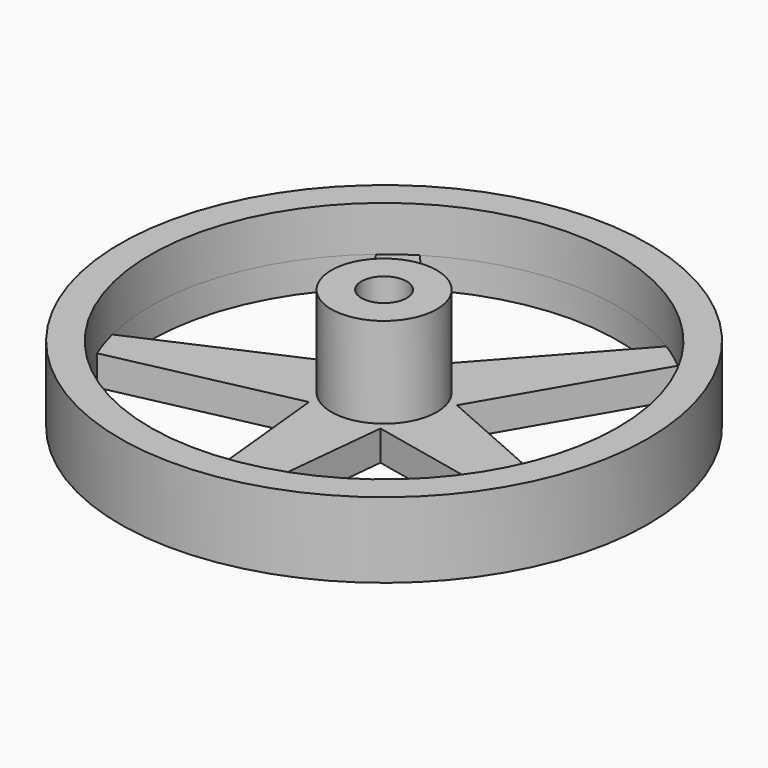
from build123d import *

# Parameters (mm, degrees)
F0_R     = 17.5
F1_DEPTH = 5
F2_R     = 15.5
F3_DEPTH = 3
F4_R     = 3.5
F4_R_2   = 1.5
F5_DEPTH = 6
F7_DEPTH = 2


with BuildPart() as f1:
    # F0 (on Top) → F1 (new body)
    with BuildSketch(Plane.XY):
        Circle(F0_R)
    extrude(amount=F1_DEPTH)

    # F2 (on face) → F3 (cut)
    with BuildSketch(Plane.XY.offset(5)):
        Circle(F2_R)
    extrude(amount=-F3_DEPTH, mode=Mode.SUBTRACT)

    # F4 (on face) → F5 (join)
    with BuildSketch(Plane.XY.offset(2)):
        Circle(F4_R)
        Circle(F4_R_2, mode=Mode.SUBTRACT)
    extrude(amount=F5_DEPTH)

    # F6 (on face) → F7 (cut)
    with BuildSketch(Plane(origin=(0, 0, 0), x_dir=(1, 0, 0), z_dir=(0, 0, -1))):
        with BuildLine():
            Line((-14.35511, 5.846437), (-2.371232, 3.263721))
            Line((-2.371232, 3.263721), (-1.124319, 15.459169))
            ThreePointArc((-1.124319, 15.459169), (-9.110671, 12.539763), (-14.35511, 5.846437))
        make_face()
        with BuildLine():
            Line((1.124319, 15.459169), (2.371232, 3.263721))
            Line((2.371232, 3.263721), (14.35511, 5.846437))
            ThreePointArc((14.35511, 5.846437), (9.110671, 12.539763), (1.124319, 15.459169))
        make_face()
        with BuildLine():
            Line((15.049977, 3.707855), (3.836734, -1.246631))
            Line((3.836734, -1.246631), (9.996265, -11.845872))
            ThreePointArc((9.996265, -11.845872), (14.056886, -6.530999), (15.5, 0))
            ThreePointArc((15.5, 0), (15.387083, 1.867532), (15.049977, 3.707855))
        make_face()
        with BuildLine():
            Line((8.177078, -13.167589), (0, -4.034181))
            Line((0, -4.034181), (-8.177078, -13.167589))
            ThreePointArc((-8.177078, -13.167589), (0, -15.5), (8.177078, -13.167589))
        make_face()
        with BuildLine():
            Line((-9.996265, -11.845872), (-3.836734, -1.246631))
            Line((-3.836734, -1.246631), (-15.049977, 3.707855))
            ThreePointArc((-15.049977, 3.707855), (-14.741376, -4.789763), (-9.996265, -11.845872))
        make_face()
    extrude(amount=-F7_DEPTH, mode=Mode.SUBTRACT)


solid = f1.part
